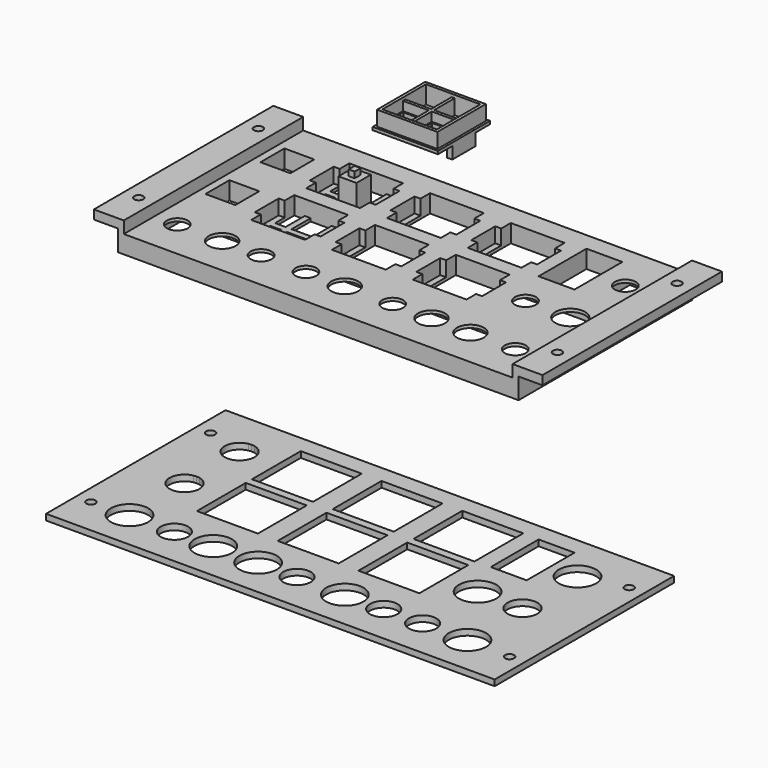
from build123d import *

# Parameters (mm, degrees)
F0_W      = 150
F0_H      = 75
F0_R      = 1.5
F0_R_2    = 3.5
F0_R_3    = 4.5
F0_R_4    = 5
F0_W_2    = 12
F0_H_2    = 20
F0_W_3    = 2
F0_H_3    = 10
F2_DEPTH  = 1
F3_DEPTH  = 5
F4_W      = 2
F4_H      = 10
F4_W_2    = 10
F5_DEPTH  = 5
F6_W      = 1.8
F6_H      = 9.8
F7_DEPTH  = 1
F8_DEPTH  = 4
F9_W      = 20.2
F9_H      = 20.2
F9_W_2    = 18.2
F9_H_2    = 18.2
F10_DEPTH = 5
F12_W     = 6
F12_H     = 4
F12_H_2   = 2
F13_DEPTH = 8
F11_W     = 8.6
F11_H     = 1
F11_W_2   = 1
F11_H_2   = 8.6
F14_DEPTH = 6
F15_W     = 18.2
F15_H     = 18.2
F16_DEPTH = 1
F18_W     = 2
F18_H     = 2.5
F19_DEPTH = 2
F20_W     = 8.6
F20_H     = 8.6
F20_W_2   = 7.6
F20_H_2   = 7.6
F21_DEPTH = 2
F17_W     = 2
F17_H     = 2.5
F22_DEPTH = 2
F23_R     = 3.5
F23_R_2   = 4.5
F23_R_3   = 5
F23_W     = 16
F23_H     = 21
F24_DEPTH = 5
F1_W      = 150
F1_H      = 75
F1_R      = 1.5
F1_R_2    = 6.25
F1_R_3    = 4.6
F1_W_2    = 20.4
F1_H_2    = 20.4
F1_R_4    = 5
F1_W_3    = 12
F1_H_3    = 20
F25_DEPTH = 2
F26_W     = 10
F26_H     = 75
F26_R     = 1.5
F27_DEPTH = 4
F28_W     = 8
F28_H     = 7
F29_DEPTH = 77.8
F30_W     = 134
F30_H     = 2.5
F31_DEPTH = 3


# Not quite as in the source:
# - a feature names something its author has since deleted; it is built from what else it names


with BuildPart() as f2:
    # F0 (on Top) → F2 (new body)
    with BuildSketch(Plane.XY):
        with Locations((-74.504784634, -19.5405644029)):
            Rectangle(F0_W, F0_H)
        with Locations((-144.504784634, -44.5405644029)):
            Circle(F0_R, mode=Mode.SUBTRACT)
        with Locations((-132.004784634, -44.0405644029)):
            Circle(F0_R_2, mode=Mode.SUBTRACT)
        with Locations((-117.004784634, -44.0405644029)):
            Circle(F0_R_3, mode=Mode.SUBTRACT)
        with Locations((-104.004784634, -44.0405644029)):
            Circle(F0_R_2, mode=Mode.SUBTRACT)
        with Locations((-89.004784634, -44.0405644029)):
            Circle(F0_R_2, mode=Mode.SUBTRACT)
        with Locations((-76.004784634, -44.0405644029)):
            Circle(F0_R_3, mode=Mode.SUBTRACT)
        Polygon((-127.004784634, -16.0405644029), (-127.004784634, -26.0405644029), (-131.004784634, -26.0405644029), (-133.004784634, -26.0405644029), (-137.004784634, -26.0405644029), (-137.004784634, -16.0405644029), (-133.004784634, -16.0405644029), (-131.004784634, -16.0405644029), align=None, mode=Mode.SUBTRACT)
        Polygon((-100.504784634, -22.0405644029), (-100.504784634, -30.0405644029), (-104.004784634, -30.0405644029), (-106.004784634, -30.0405644029), (-113.004784634, -30.0405644029), (-115.004784634, -30.0405644029), (-118.504784634, -30.0405644029), (-118.504784634, -22.0405644029), (-118.504784634, -20.0405644029), (-118.504784634, -12.0405644029), (-115.004784634, -12.0405644029), (-113.004784634, -12.0405644029), (-106.004784634, -12.0405644029), (-104.004784634, -12.0405644029), (-100.504784634, -12.0405644029), (-100.504784634, -20.0405644029), align=None, mode=Mode.SUBTRACT)
        Polygon((-77.004784634, -30.0405644029), (-79.004784634, -30.0405644029), (-86.004784634, -30.0405644029), (-88.004784634, -30.0405644029), (-91.504784634, -30.0405644029), (-91.504784634, -22.0405644029), (-91.504784634, -20.0405644029), (-91.504784634, -12.0405644029), (-88.004784634, -12.0405644029), (-86.004784634, -12.0405644029), (-79.004784634, -12.0405644029), (-77.004784634, -12.0405644029), (-73.504784634, -12.0405644029), (-73.504784634, -20.0405644029), (-73.504784634, -22.0405644029), (-73.504784634, -30.0405644029), align=None, mode=Mode.SUBTRACT)
        with Locations((-60.004784634, -44.0405644029)):
            Circle(F0_R_2, mode=Mode.SUBTRACT)
        with Locations((-47.004784634, -44.0405644029)):
            Circle(F0_R_3, mode=Mode.SUBTRACT)
        with Locations((-34.004784634, -44.0405644029)):
            Circle(F0_R_3, mode=Mode.SUBTRACT)
        with Locations((-19.004784634, -44.0405644029)):
            Circle(F0_R_2, mode=Mode.SUBTRACT)
        with Locations((-4.504784634, -44.5405644029)):
            Circle(F0_R, mode=Mode.SUBTRACT)
        Polygon((-50.004784634, -30.0405644029), (-52.004784634, -30.0405644029), (-59.004784634, -30.0405644029), (-61.004784634, -30.0405644029), (-64.504784634, -30.0405644029), (-64.504784634, -22.0405644029), (-64.504784634, -20.0405644029), (-64.504784634, -12.0405644029), (-61.004784634, -12.0405644029), (-59.004784634, -12.0405644029), (-52.004784634, -12.0405644029), (-50.004784634, -12.0405644029), (-46.504784634, -12.0405644029), (-46.504784634, -20.0405644029), (-46.504784634, -22.0405644029), (-46.504784634, -30.0405644029), align=None, mode=Mode.SUBTRACT)
        with Locations((-34.004784634, -21.0405644029)):
            Circle(F0_R_2, mode=Mode.SUBTRACT)
        with Locations((-19.004784634, -21.0405644029)):
            Circle(F0_R_4, mode=Mode.SUBTRACT)
        Polygon((-127.004784634, 6.9594355971), (-127.004784634, -3.0405644029), (-131.004784634, -3.0405644029), (-133.004784634, -3.0405644029), (-137.004784634, -3.0405644029), (-137.004784634, 6.9594355971), (-133.004784634, 6.9594355971), (-131.004784634, 6.9594355971), align=None, mode=Mode.SUBTRACT)
        with Locations((-144.504784634, 5.4594355971)):
            Circle(F0_R, mode=Mode.SUBTRACT)
        Polygon((-100.504784634, 0.9594355971), (-100.504784634, -7.0405644029), (-104.004784634, -7.0405644029), (-106.004784634, -7.0405644029), (-113.004784634, -7.0405644029), (-115.004784634, -7.0405644029), (-118.504784634, -7.0405644029), (-118.504784634, 0.9594355971), (-118.504784634, 2.9594355971), (-118.504784634, 10.9594355971), (-115.004784634, 10.9594355971), (-113.004784634, 10.9594355971), (-106.004784634, 10.9594355971), (-104.004784634, 10.9594355971), (-100.504784634, 10.9594355971), (-100.504784634, 2.9594355971), align=None, mode=Mode.SUBTRACT)
        Polygon((-73.504784634, 10.9594355971), (-73.504784634, 2.9594355971), (-73.504784634, 0.9594355971), (-73.504784634, -7.0405644029), (-77.004784634, -7.0405644029), (-79.004784634, -7.0405644029), (-86.004784634, -7.0405644029), (-88.004784634, -7.0405644029), (-91.504784634, -7.0405644029), (-91.504784634, 0.9594355971), (-91.504784634, 2.9594355971), (-91.504784634, 10.9594355971), (-88.004784634, 10.9594355971), (-86.004784634, 10.9594355971), (-79.004784634, 10.9594355971), (-77.004784634, 10.9594355971), align=None, mode=Mode.SUBTRACT)
        Polygon((-46.504784634, 10.9594355971), (-46.504784634, 2.9594355971), (-46.504784634, 0.9594355971), (-46.504784634, -7.0405644029), (-50.004784634, -7.0405644029), (-52.004784634, -7.0405644029), (-59.004784634, -7.0405644029), (-61.004784634, -7.0405644029), (-64.504784634, -7.0405644029), (-64.504784634, 0.9594355971), (-64.504784634, 2.9594355971), (-64.504784634, 10.9594355971), (-61.004784634, 10.9594355971), (-59.004784634, 10.9594355971), (-52.004784634, 10.9594355971), (-50.004784634, 10.9594355971), align=None, mode=Mode.SUBTRACT)
        with Locations((-34.004784634, 1.9594355971)):
            Rectangle(F0_W_2, F0_H_2, mode=Mode.SUBTRACT)
        with Locations((-19.004784634, 1.9594355971)):
            Circle(F0_R_2, mode=Mode.SUBTRACT)
        with Locations((-4.504784634, 5.4594355971)):
            Circle(F0_R, mode=Mode.SUBTRACT)
        Polygon((-106.004784634, -7.0405644029), (-104.004784634, -7.0405644029), (-104.004784634, 0.9594355971), (-100.504784634, 0.9594355971), (-100.504784634, 2.9594355971), (-104.004784634, 2.9594355971), (-104.004784634, 10.9594355971), (-106.004784634, 10.9594355971), (-106.004784634, 2.9594355971), (-113.004784634, 2.9594355971), (-113.004784634, 10.9594355971), (-115.004784634, 10.9594355971), (-115.004784634, 2.9594355971), (-118.504784634, 2.9594355971), (-118.504784634, 0.9594355971), (-115.004784634, 0.9594355971), (-115.004784634, -7.0405644029), (-113.004784634, -7.0405644029), (-113.004784634, 0.9594355971), (-106.004784634, 0.9594355971), align=None)
        Polygon((-106.004784634, -30.0405644029), (-104.004784634, -30.0405644029), (-104.004784634, -22.0405644029), (-100.504784634, -22.0405644029), (-100.504784634, -20.0405644029), (-104.004784634, -20.0405644029), (-104.004784634, -12.0405644029), (-106.004784634, -12.0405644029), (-106.004784634, -20.0405644029), (-113.004784634, -20.0405644029), (-113.004784634, -12.0405644029), (-115.004784634, -12.0405644029), (-115.004784634, -20.0405644029), (-118.504784634, -20.0405644029), (-118.504784634, -22.0405644029), (-115.004784634, -22.0405644029), (-115.004784634, -30.0405644029), (-113.004784634, -30.0405644029), (-113.004784634, -22.0405644029), (-106.004784634, -22.0405644029), align=None)
        with Locations((-132.004784634, 1.9594355971)):
            Rectangle(F0_W_3, F0_H_3)
        with Locations((-132.004784634, -21.0405644029)):
            Rectangle(F0_W_3, F0_H_3)
    extrude(amount=F2_DEPTH)

    # F3 (add): a face of the model
    f3_faces = [f2.faces().sort_by_distance(p)[0] for p in [
        (-1.1818356172, -19.5405644029, 1),
    ]]
    extrude(f3_faces, amount=F3_DEPTH)

    # F4 (on face) → F5 (cut)
    with BuildSketch(Plane.XY.offset(6)):
        Polygon((-118.504784634, -7.0405644029), (-100.504784634, -7.0405644029), (-100.504784634, -3.0405644029), (-100.504784634, 6.9594355971), (-100.504784634, 10.9594355971), (-118.504784634, 10.9594355971), (-118.504784634, 6.9594355971), (-118.504784634, -3.0405644029), align=None)
        with Locations((-99.504784634, 1.9594355971)):
            Rectangle(F4_W, F4_H)
        with Locations((-119.504784634, 1.9594355971)):
            Rectangle(F4_W, F4_H)
        Polygon((-118.504784634, -30.0405644029), (-100.504784634, -30.0405644029), (-100.504784634, -26.0405644029), (-100.504784634, -16.0405644029), (-100.504784634, -12.0405644029), (-118.504784634, -12.0405644029), (-118.504784634, -16.0405644029), (-118.504784634, -26.0405644029), align=None)
        with Locations((-99.504784634, -21.0405644029)):
            Rectangle(F4_W, F4_H)
        with Locations((-119.504784634, -21.0405644029)):
            Rectangle(F4_W, F4_H)
        with Locations((-72.504784634, 1.9594355971)):
            Rectangle(F4_W, F4_H)
        Polygon((-73.504784634, -7.0405644029), (-73.504784634, -3.0405644029), (-73.504784634, 6.9594355971), (-73.504784634, 10.9594355971), (-91.504784634, 10.9594355971), (-91.504784634, 6.9594355971), (-91.504784634, -3.0405644029), (-91.504784634, -7.0405644029), align=None)
        with Locations((-92.504784634, 1.9594355971)):
            Rectangle(F4_W, F4_H)
        with Locations((-45.504784634, 1.9594355971)):
            Rectangle(F4_W, F4_H)
        Polygon((-46.504784634, -7.0405644029), (-46.504784634, -3.0405644029), (-46.504784634, 6.9594355971), (-46.504784634, 10.9594355971), (-64.504784634, 10.9594355971), (-64.504784634, 6.9594355971), (-64.504784634, -3.0405644029), (-64.504784634, -7.0405644029), align=None)
        with Locations((-65.504784634, 1.9594355971)):
            Rectangle(F4_W, F4_H)
        with Locations((-72.504784634, -21.0405644029)):
            Rectangle(F4_W, F4_H)
        Polygon((-73.504784634, -26.0405644029), (-73.504784634, -16.0405644029), (-73.504784634, -12.0405644029), (-91.504784634, -12.0405644029), (-91.504784634, -16.0405644029), (-91.504784634, -26.0405644029), (-91.504784634, -30.0405644029), (-73.504784634, -30.0405644029), align=None)
        with Locations((-92.504784634, -21.0405644029)):
            Rectangle(F4_W, F4_H)
        with Locations((-45.504784634, -21.0405644029)):
            Rectangle(F4_W, F4_H)
        Polygon((-46.504784634, -26.0405644029), (-46.504784634, -16.0405644029), (-46.504784634, -12.0405644029), (-64.504784634, -12.0405644029), (-64.504784634, -16.0405644029), (-64.504784634, -26.0405644029), (-64.504784634, -30.0405644029), (-46.504784634, -30.0405644029), align=None)
        with Locations((-65.504784634, -21.0405644029)):
            Rectangle(F4_W, F4_H)
        with Locations((-132.004784634, 1.9594355971)):
            Rectangle(F4_W_2, F4_H)
        with Locations((-132.004784634, -21.0405644029)):
            Rectangle(F4_W_2, F4_H)
    extrude(amount=-F5_DEPTH, mode=Mode.SUBTRACT)

    # F12 (on face) → F13 (join)
    with BuildSketch(Plane.XY.offset(1)):
        with Locations((-109.504784634, 2.9594355971)):
            Rectangle(F12_W, F12_H)
        with Locations((-109.504784634, -0.0405644029)):
            Rectangle(F12_W, F12_H_2)
    extrude(amount=F13_DEPTH)

    # F18 (on face) → F19 (join)
    with BuildSketch(Plane.XY.offset(9)):
        with Locations((-109.504784634, 1.9594355971)):
            Rectangle(F18_W, F18_H)
    extrude(amount=F19_DEPTH)

    # F23 (on face) → F24 (cut)
    with BuildSketch(Plane.XY):
        Polygon((-43.504784634, -33.0405644029), (-139.504784634, -33.0405644029), (-139.504784634, -55.0405644029), (-9.504784634, -55.0405644029), (-9.504784634, -33.0405644029), align=None)
        with Locations((-132.004784634, -44.0405644029)):
            Circle(F23_R, mode=Mode.SUBTRACT)
        with Locations((-117.004784634, -44.0405644029)):
            Circle(F23_R_2, mode=Mode.SUBTRACT)
        with Locations((-104.004784634, -44.0405644029)):
            Circle(F23_R, mode=Mode.SUBTRACT)
        with Locations((-89.004784634, -44.0405644029)):
            Circle(F23_R, mode=Mode.SUBTRACT)
        with Locations((-76.004784634, -44.0405644029)):
            Circle(F23_R_2, mode=Mode.SUBTRACT)
        with Locations((-60.004784634, -44.0405644029)):
            Circle(F23_R, mode=Mode.SUBTRACT)
        with Locations((-47.004784634, -44.0405644029)):
            Circle(F23_R_2, mode=Mode.SUBTRACT)
        with Locations((-34.004784634, -44.0405644029)):
            Circle(F23_R_2, mode=Mode.SUBTRACT)
        with Locations((-19.004784634, -44.0405644029)):
            Circle(F23_R, mode=Mode.SUBTRACT)
        Polygon((-43.504784634, -11.0405644029), (-43.504784634, -31.0405644029), (-9.504784634, -31.0405644029), (-9.504784634, -11.0405644029), (-25.504784634, -11.0405644029), align=None)
        with Locations((-34.004784634, -21.0405644029)):
            Circle(F23_R, mode=Mode.SUBTRACT)
        with Locations((-19.004784634, -21.0405644029)):
            Circle(F23_R_3, mode=Mode.SUBTRACT)
        with Locations((-17.504784634, 1.4594355971)):
            Rectangle(F23_W, F23_H)
        with Locations((-19.004784634, 1.9594355971)):
            Circle(F23_R, mode=Mode.SUBTRACT)
        with Locations((-19.004784634, -21.0405644029)):
            Circle(F23_R_3)
        with Locations((-117.004784634, -44.0405644029)):
            Circle(F23_R_2)
        with Locations((-76.004784634, -44.0405644029)):
            Circle(F23_R_2)
        with Locations((-47.004784634, -44.0405644029)):
            Circle(F23_R_2)
        with Locations((-34.004784634, -44.0405644029)):
            Circle(F23_R_2)
        with Locations((-132.004784634, -44.0405644029)):
            Circle(F23_R)
        with Locations((-104.004784634, -44.0405644029)):
            Circle(F23_R)
        with Locations((-89.004784634, -44.0405644029)):
            Circle(F23_R)
        with Locations((-60.004784634, -44.0405644029)):
            Circle(F23_R)
        with Locations((-19.004784634, -44.0405644029)):
            Circle(F23_R)
        with Locations((-34.004784634, -21.0405644029)):
            Circle(F23_R)
        with Locations((-19.004784634, 1.9594355971)):
            Circle(F23_R)
    extrude(amount=F24_DEPTH, mode=Mode.SUBTRACT)

    # F26 (on face) → F27 (join)
    with BuildSketch(Plane.XY.offset(6)):
        with Locations((-4.504784634, -19.5405644029)):
            Rectangle(F26_W, F26_H)
        with Locations((-4.504784634, -44.5405644029)):
            Circle(F26_R, mode=Mode.SUBTRACT)
        with Locations((-4.504784634, 5.4594355971)):
            Circle(F26_R, mode=Mode.SUBTRACT)
        with Locations((-144.504784634, -19.5405644029)):
            Rectangle(F26_W, F26_H)
        with Locations((-144.504784634, -44.5405644029)):
            Circle(F26_R, mode=Mode.SUBTRACT)
        with Locations((-144.504784634, 5.4594355971)):
            Circle(F26_R, mode=Mode.SUBTRACT)
    extrude(amount=F27_DEPTH)

    # F28 (on face) → F29 (cut)
    with BuildSketch(Plane.XZ.offset(57.0405644029)):
        with Locations((-145.504784634, 3.5)):
            Rectangle(F28_W, F28_H)
        with Locations((-3.504784634, 3.5)):
            Rectangle(F28_W, F28_H)
    extrude(amount=-F29_DEPTH, mode=Mode.SUBTRACT)

    # F30 (on face) → F31 (cut)
    with BuildSketch(Plane(origin=(0, 0, 0), x_dir=(1, 0, 0), z_dir=(0, 0, -1))):
        with Locations((-74.504784634, -16.7094355971)):
            Rectangle(F30_W, F30_H)
    extrude(amount=-F31_DEPTH, mode=Mode.SUBTRACT)


with BuildPart() as f7:
    # F6 (on Top) → F7 (new body)
    with BuildSketch(Plane.XY):
        Polygon((-132.6183355093, 38.3936729491), (-110.8183355093, 38.3936729491), (-110.8183355093, 44.3936729491), (-112.6183355093, 44.3936729491), (-112.6183355093, 40.1936729491), (-130.8183355093, 40.1936729491), (-130.8183355093, 44.3936729491), (-132.6183355093, 44.3936729491), align=None)
        with Locations((-111.7183355093, 49.2936729491)):
            Rectangle(F6_W, F6_H)
        with Locations((-131.7183355093, 49.2936729491)):
            Rectangle(F6_W, F6_H)
        Polygon((-112.6183355093, 54.1936729491), (-110.8183355093, 54.1936729491), (-110.8183355093, 60.1936729491), (-132.6183355093, 60.1936729491), (-132.6183355093, 54.1936729491), (-130.8183355093, 54.1936729491), (-130.8183355093, 58.3936729491), (-112.6183355093, 58.3936729491), align=None)
    extrude(amount=F7_DEPTH)

    # F6 (on Top) → F8 (join)
    with BuildSketch(Plane.XY):
        with Locations((-131.7183355093, 49.2936729491)):
            Rectangle(F6_W, F6_H)
        with Locations((-111.7183355093, 49.2936729491)):
            Rectangle(F6_W, F6_H)
    extrude(amount=-F8_DEPTH)

    # F9 (on face) → F10 (join)
    with BuildSketch(Plane.XY.offset(1)):
        with Locations((-121.7183355093, 49.2936729491)):
            Rectangle(F9_W, F9_H)
        with Locations((-121.7183355093, 49.2936729491)):
            Rectangle(F9_W_2, F9_H_2, mode=Mode.SUBTRACT)
    extrude(amount=F10_DEPTH)

    # F11 (on face) → F14 (join)
    with BuildSketch(Plane.XY.offset(6)):
        with Locations((-116.9183355093, 49.2936729491)):
            Rectangle(F11_W, F11_H)
        with Locations((-121.7183355093, 44.4936729491)):
            Rectangle(F11_W_2, F11_H_2)
        with Locations((-121.7183355093, 49.2936729491)):
            Rectangle(F11_W_2, F11_H)
        with Locations((-126.5183355093, 49.2936729491)):
            Rectangle(F11_W, F11_H)
        with Locations((-121.7183355093, 54.0936729491)):
            Rectangle(F11_W_2, F11_H_2)
    extrude(amount=-F14_DEPTH)

    # F15 (on face) → F16 (cut)
    with BuildSketch(Plane.XY.offset(6)):
        with Locations((-121.7183355093, 49.2936729491)):
            Rectangle(F15_W, F15_H)
    extrude(amount=-F16_DEPTH, mode=Mode.SUBTRACT)

    # F20 (on face) → F21 (join)
    with BuildSketch(Plane(origin=(0, 0, 0), x_dir=(1, 0, 0), z_dir=(0, 0, -1))):
        with Locations((-126.5183355093, -44.4936729491)):
            Rectangle(F20_W, F20_H)
        with Locations((-126.5183355093, -44.4936729491)):
            Rectangle(F20_W_2, F20_H_2, mode=Mode.SUBTRACT)
        with Locations((-116.9183355093, -44.4936729491)):
            Rectangle(F20_W, F20_H)
        with Locations((-116.9183355093, -44.4936729491)):
            Rectangle(F20_W_2, F20_H_2, mode=Mode.SUBTRACT)
    extrude(amount=-F21_DEPTH)

    # F17 (on face) → F22 (cut)
    with BuildSketch(Plane(origin=(0, 0, 0), x_dir=(1, 0, 0), z_dir=(0, 0, -1))):
        with Locations((-121.7183355093, -49.2936729491)):
            Rectangle(F17_W, F17_H)
    extrude(amount=-F22_DEPTH, mode=Mode.SUBTRACT)


with BuildPart() as f25:
    # F1 (on Top) → F25 (new body)
    with BuildSketch(Plane.XY):
        with Locations((13.6568725579, -149.7262832487)):
            Rectangle(F1_W, F1_H)
        with Locations((-56.3431274421, -174.7262832487)):
            Circle(F1_R, mode=Mode.SUBTRACT)
        with Locations((-43.8431274421, -174.2262832487)):
            Circle(F1_R_2, mode=Mode.SUBTRACT)
        with Locations((-28.8431274421, -174.2262832487)):
            Circle(F1_R_3, mode=Mode.SUBTRACT)
        with Locations((-15.8431274421, -174.2262832487)):
            Circle(F1_R_2, mode=Mode.SUBTRACT)
        with Locations((-0.8431274421, -174.2262832487)):
            Circle(F1_R_2, mode=Mode.SUBTRACT)
        with Locations((12.1568725579, -174.2262832487)):
            Circle(F1_R_3, mode=Mode.SUBTRACT)
        with BuildLine():
            Line((-42.8431274421, -156.1252627342), (-42.8431274421, -156.2262832487))
            Line((-42.8431274421, -156.2262832487), (-43.8431274421, -156.2262832487))
            Line((-43.8431274421, -156.2262832487), (-44.8431274421, -156.2262832487))
            Line((-44.8431274421, -156.2262832487), (-44.8431274421, -156.1252627342))
            ThreePointArc((-44.8431274421, -156.1252627342), (-48.8431274421, -151.2262832487), (-44.8431274421, -146.3273037631))
            Line((-44.8431274421, -146.3273037631), (-44.8431274421, -146.2262832487))
            Line((-44.8431274421, -146.2262832487), (-43.8431274421, -146.2262832487))
            Line((-43.8431274421, -146.2262832487), (-42.8431274421, -146.2262832487))
            Line((-42.8431274421, -146.2262832487), (-42.8431274421, -146.3273037631))
            ThreePointArc((-42.8431274421, -146.3273037631), (-39.9701440959, -148.0640055885), (-38.8431274421, -151.2262832487))
            ThreePointArc((-38.8431274421, -151.2262832487), (-39.9701440959, -154.3885609088), (-42.8431274421, -156.1252627342))
        make_face(mode=Mode.SUBTRACT)
        with Locations((-21.3431274421, -151.2262832487)):
            Rectangle(F1_W_2, F1_H_2, mode=Mode.SUBTRACT)
        with Locations((5.6568725579, -151.2262832487)):
            Rectangle(F1_W_2, F1_H_2, mode=Mode.SUBTRACT)
        with Locations((28.1568725579, -174.2262832487)):
            Circle(F1_R_2, mode=Mode.SUBTRACT)
        with Locations((41.1568725579, -174.2262832487)):
            Circle(F1_R_3, mode=Mode.SUBTRACT)
        with Locations((54.1568725579, -174.2262832487)):
            Circle(F1_R_3, mode=Mode.SUBTRACT)
        with Locations((69.1568725579, -174.2262832487)):
            Circle(F1_R_2, mode=Mode.SUBTRACT)
        with Locations((83.6568725579, -174.7262832487)):
            Circle(F1_R, mode=Mode.SUBTRACT)
        with Locations((32.6568725579, -151.2262832487)):
            Rectangle(F1_W_2, F1_H_2, mode=Mode.SUBTRACT)
        with Locations((54.1568725579, -151.2262832487)):
            Circle(F1_R_2, mode=Mode.SUBTRACT)
        with Locations((69.1568725579, -151.2262832487)):
            Circle(F1_R_4, mode=Mode.SUBTRACT)
        with BuildLine():
            Line((-42.8431274421, -133.1252627342), (-42.8431274421, -133.2262832487))
            Line((-42.8431274421, -133.2262832487), (-43.8431274421, -133.2262832487))
            Line((-43.8431274421, -133.2262832487), (-44.8431274421, -133.2262832487))
            Line((-44.8431274421, -133.2262832487), (-44.8431274421, -133.1252627342))
            ThreePointArc((-44.8431274421, -133.1252627342), (-48.8431274421, -128.2262832487), (-44.8431274421, -123.3273037631))
            Line((-44.8431274421, -123.3273037631), (-44.8431274421, -123.2262832487))
            Line((-44.8431274421, -123.2262832487), (-43.8431274421, -123.2262832487))
            Line((-43.8431274421, -123.2262832487), (-42.8431274421, -123.2262832487))
            Line((-42.8431274421, -123.2262832487), (-42.8431274421, -123.3273037631))
            ThreePointArc((-42.8431274421, -123.3273037631), (-39.9701440959, -125.0640055885), (-38.8431274421, -128.2262832487))
            ThreePointArc((-38.8431274421, -128.2262832487), (-39.9701440959, -131.3885609088), (-42.8431274421, -133.1252627342))
        make_face(mode=Mode.SUBTRACT)
        with Locations((-56.3431274421, -124.7262832487)):
            Circle(F1_R, mode=Mode.SUBTRACT)
        with Locations((-21.3431274421, -128.2262832487)):
            Rectangle(F1_W_2, F1_H_2, mode=Mode.SUBTRACT)
        with Locations((5.6568725579, -128.2262832487)):
            Rectangle(F1_W_2, F1_H_2, mode=Mode.SUBTRACT)
        with Locations((32.6568725579, -128.2262832487)):
            Rectangle(F1_W_2, F1_H_2, mode=Mode.SUBTRACT)
        with Locations((54.1568725579, -128.2262832487)):
            Rectangle(F1_W_3, F1_H_3, mode=Mode.SUBTRACT)
        with Locations((69.1568725579, -128.2262832487)):
            Circle(F1_R_2, mode=Mode.SUBTRACT)
        with Locations((83.6568725579, -124.7262832487)):
            Circle(F1_R, mode=Mode.SUBTRACT)
        with BuildLine():
            Line((-44.8431274421, -146.2262832487), (-44.8431274421, -146.3273037631))
            ThreePointArc((-44.8431274421, -146.3273037631), (-44.3456722522, -146.2516024836), (-43.8431274421, -146.2262832487))
            Line((-43.8431274421, -146.2262832487), (-44.8431274421, -146.2262832487))
        make_face()
        with BuildLine():
            ThreePointArc((-43.8431274421, -146.2262832487), (-43.3405826321, -146.2516024836), (-42.8431274421, -146.3273037631))
            Line((-42.8431274421, -146.3273037631), (-42.8431274421, -146.2262832487))
            Line((-42.8431274421, -146.2262832487), (-43.8431274421, -146.2262832487))
        make_face()
        with BuildLine():
            Line((-44.8431274421, -156.2262832487), (-43.8431274421, -156.2262832487))
            ThreePointArc((-43.8431274421, -156.2262832487), (-44.3456722522, -156.2009640137), (-44.8431274421, -156.1252627342))
            Line((-44.8431274421, -156.1252627342), (-44.8431274421, -156.2262832487))
        make_face()
        with BuildLine():
            Line((-43.8431274421, -156.2262832487), (-42.8431274421, -156.2262832487))
            Line((-42.8431274421, -156.2262832487), (-42.8431274421, -156.1252627342))
            ThreePointArc((-42.8431274421, -156.1252627342), (-43.3405826321, -156.2009640137), (-43.8431274421, -156.2262832487))
        make_face()
        with BuildLine():
            Line((-44.8431274421, -123.2262832487), (-44.8431274421, -123.3273037631))
            ThreePointArc((-44.8431274421, -123.3273037631), (-44.3456722522, -123.2516024836), (-43.8431274421, -123.2262832487))
            Line((-43.8431274421, -123.2262832487), (-44.8431274421, -123.2262832487))
        make_face()
        with BuildLine():
            ThreePointArc((-43.8431274421, -123.2262832487), (-43.3405826321, -123.2516024836), (-42.8431274421, -123.3273037631))
            Line((-42.8431274421, -123.3273037631), (-42.8431274421, -123.2262832487))
            Line((-42.8431274421, -123.2262832487), (-43.8431274421, -123.2262832487))
        make_face()
        with BuildLine():
            Line((-44.8431274421, -133.2262832487), (-43.8431274421, -133.2262832487))
            ThreePointArc((-43.8431274421, -133.2262832487), (-44.3456722522, -133.2009640137), (-44.8431274421, -133.1252627342))
            Line((-44.8431274421, -133.1252627342), (-44.8431274421, -133.2262832487))
        make_face()
        with BuildLine():
            Line((-43.8431274421, -133.2262832487), (-42.8431274421, -133.2262832487))
            Line((-42.8431274421, -133.2262832487), (-42.8431274421, -133.1252627342))
            ThreePointArc((-42.8431274421, -133.1252627342), (-43.3405826321, -133.2009640137), (-43.8431274421, -133.2262832487))
        make_face()
    extrude(amount=F25_DEPTH)


solid = Compound([f2.part, f7.part, f25.part])
